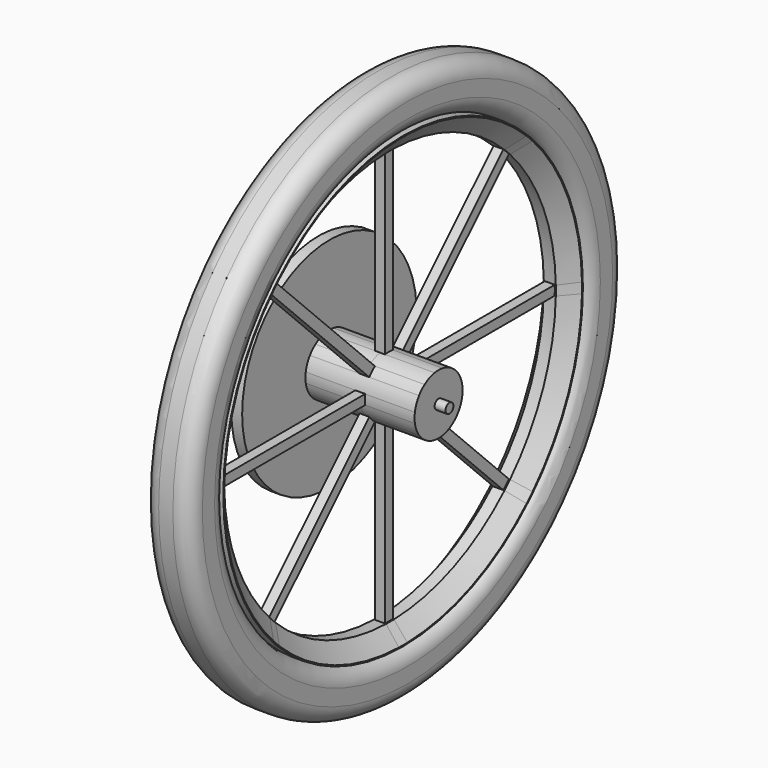
from build123d import *

# Parameters (mm, degrees)
F0_R       = 4.5
F1_DEPTH   = 60
F2_DEPTH   = 50
F3_DEPTH   = 4.5
F0_R_2     = 250
F0_R_3     = 206
F4_DEPTH   = 21.5
F5_DEPTH   = 17.5
F6_R       = 15
F7_SIZE2   = 12
F7_SIZE    = 15
F7_2_SIZE2 = 12
F7_2_SIZE  = 15
F8_R       = 100
F9_DEPTH   = 10
F10_R      = 4.5
F11_DEPTH  = 15


# Not quite as in the source:
# - a feature names something its author has since deleted; it is built from what else it names


with BuildPart() as f1:
    # F0 (on Right) → F1 (new body, symmetric)
    with BuildSketch(Plane.YZ):
        Circle(F0_R)
    extrude(amount=F1_DEPTH, both=True)

    # F0 (on Right) → F2 (join, symmetric)
    with BuildSketch(Plane.YZ):
        with BuildLine():
            ThreePointArc((27.5, 0), (27.4146857974, 2.1644866893), (27.1592725361, 4.3155434546))
            ThreePointArc((27.1592725361, 4.3155434546), (25.4422970206, 10.4374097514), (22.3653066086, 16.0013455779))
            ThreePointArc((22.3653066086, 16.0013455779), (19.4454364826, 19.4454364826), (16.0013455779, 22.3653066086))
            ThreePointArc((16.0013455779, 22.3653066086), (10.52379439, 25.4066871441), (4.5, 27.1293199325))
            ThreePointArc((4.5, 27.1293199325), (0, 27.5), (-4.5, 27.1293199325))
            ThreePointArc((-4.5, 27.1293199325), (-10.52379439, 25.4066871441), (-16.0013455779, 22.3653066086))
            ThreePointArc((-16.0013455779, 22.3653066086), (-19.4454364826, 19.4454364826), (-22.3653066086, 16.0013455779))
            ThreePointArc((-22.3653066086, 16.0013455779), (-25.4066871441, 10.52379439), (-27.1293199325, 4.5))
            ThreePointArc((-27.1293199325, 4.5), (-27.5, 0), (-27.1293199325, -4.5))
            ThreePointArc((-27.1293199325, -4.5), (-25.4066871441, -10.52379439), (-22.3653066086, -16.0013455779))
            ThreePointArc((-22.3653066086, -16.0013455779), (-19.4454364826, -19.4454364826), (-16.0013455779, -22.3653066086))
            ThreePointArc((-16.0013455779, -22.3653066086), (-10.52379439, -25.4066871441), (-4.5, -27.1293199325))
            ThreePointArc((-4.5, -27.1293199325), (0, -27.5), (4.5, -27.1293199325))
            ThreePointArc((4.5, -27.1293199325), (10.52379439, -25.4066871441), (16.0013455779, -22.3653066086))
            ThreePointArc((16.0013455779, -22.3653066086), (19.4454364826, -19.4454364826), (22.3653066086, -16.0013455779))
            ThreePointArc((22.3653066086, -16.0013455779), (25.4066871441, -10.52379439), (27.1293199325, -4.5))
            ThreePointArc((27.1293199325, -4.5), (27.4071733142, -2.2576206342), (27.5, 0))
        make_face()
        Circle(F0_R, mode=Mode.SUBTRACT)
    extrude(amount=F2_DEPTH, both=True)

    # F0 (on Right) → F3 (join, symmetric)
    with BuildSketch(Plane.YZ):
        with BuildLine():
            Line((4.5, 27.1293199325), (4.5, 189.9467030511))
            ThreePointArc((4.5, 189.9467030511), (0, 190), (-4.5, 189.9467030511))
            Line((-4.5, 189.9467030511), (-4.5, 27.1293199325))
            ThreePointArc((-4.5, 27.1293199325), (0, 27.5), (4.5, 27.1293199325))
        make_face()
        with BuildLine():
            Line((-16.0013455779, 22.3653066086), (-131.1306212762, 137.4945823068))
            ThreePointArc((-131.1306212762, 137.4945823068), (-134.3502884254, 134.3502884254), (-137.4945823068, 131.1306212762))
            Line((-137.4945823068, 131.1306212762), (-22.3653066086, 16.0013455779))
            ThreePointArc((-22.3653066086, 16.0013455779), (-19.4454364826, 19.4454364826), (-16.0013455779, 22.3653066086))
        make_face()
        with BuildLine():
            Line((-27.1293199325, 4.5), (-189.9467030511, 4.5))
            ThreePointArc((-189.9467030511, 4.5), (-190, 0), (-189.9467030511, -4.5))
            Line((-189.9467030511, -4.5), (-27.1293199325, -4.5))
            ThreePointArc((-27.1293199325, -4.5), (-27.5, 0), (-27.1293199325, 4.5))
        make_face()
        with BuildLine():
            ThreePointArc((-137.4945823068, -131.1306212762), (-134.3502884254, -134.3502884254), (-131.1306212762, -137.4945823068))
            Line((-131.1306212762, -137.4945823068), (-16.0013455779, -22.3653066086))
            ThreePointArc((-16.0013455779, -22.3653066086), (-19.4454364826, -19.4454364826), (-22.3653066086, -16.0013455779))
            Line((-22.3653066086, -16.0013455779), (-137.4945823068, -131.1306212762))
        make_face()
        with BuildLine():
            Line((22.3653066086, 16.0013455779), (137.4945823068, 131.1306212762))
            ThreePointArc((137.4945823068, 131.1306212762), (134.3502884254, 134.3502884254), (131.1306212762, 137.4945823068))
            Line((131.1306212762, 137.4945823068), (16.0013455779, 22.3653066086))
            ThreePointArc((16.0013455779, 22.3653066086), (19.4454364826, 19.4454364826), (22.3653066086, 16.0013455779))
        make_face()
        with BuildLine():
            ThreePointArc((131.1306212762, -137.4945823068), (134.3502884254, -134.3502884254), (137.4945823068, -131.1306212762))
            Line((137.4945823068, -131.1306212762), (22.3653066086, -16.0013455779))
            ThreePointArc((22.3653066086, -16.0013455779), (19.4454364826, -19.4454364826), (16.0013455779, -22.3653066086))
            Line((16.0013455779, -22.3653066086), (131.1306212762, -137.4945823068))
        make_face()
        with BuildLine():
            ThreePointArc((-4.5, -189.9467030511), (0, -190), (4.5, -189.9467030511))
            Line((4.5, -189.9467030511), (4.5, -27.1293199325))
            ThreePointArc((4.5, -27.1293199325), (0, -27.5), (-4.5, -27.1293199325))
            Line((-4.5, -27.1293199325), (-4.5, -189.9467030511))
        make_face()
        with BuildLine():
            ThreePointArc((189.9467030511, -4.5), (189.9866752956, -2.2501578036), (190, 0))
            ThreePointArc((190, 0), (189.9877454483, 2.1579109074), (189.9509833738, 4.3155434546))
            Line((189.9509833738, 4.3155434546), (27.1592725361, 4.3155434546))
            ThreePointArc((27.1592725361, 4.3155434546), (27.4146857974, 2.1644866893), (27.5, 0))
            ThreePointArc((27.5, 0), (27.4071733142, -2.2576206342), (27.1293199325, -4.5))
            Line((27.1293199325, -4.5), (189.9467030511, -4.5))
        make_face()
    extrude(amount=F3_DEPTH, both=True)

    # F8 (on face) → F9 (join)
    with BuildSketch(Plane(origin=(-50, 0, 0), x_dir=(0, -1, 0), z_dir=(-1, 0, 0))):
        Circle(F8_R)
    extrude(amount=F9_DEPTH)

    # F10 (on face) → F11 (join)
    with BuildSketch(Plane(origin=(-60, 0, 0), x_dir=(0, -1, 0), z_dir=(-1, 0, 0))):
        Circle(F10_R)
    extrude(amount=F11_DEPTH)


with BuildPart() as f4:
    # F0 (on Right) → F4 (new body, symmetric)
    with BuildSketch(Plane.YZ):
        Circle(F0_R_2)
        Circle(F0_R_3, mode=Mode.SUBTRACT)
    extrude(amount=F4_DEPTH, both=True)

    # F6
    f6_edges = [f4.edges().sort_by_distance(p)[0] for p in [
        (-21.5, -250, 0),
        (0, 250, 0),
        (21.5, -250, 0),
        (-21.5, -206, 0),
        (21.5, -206, 0),
    ]]
    fillet(f6_edges, radius=F6_R)


with BuildPart() as f5:
    # F0 (on Right) → F5 (new body, symmetric)
    with BuildSketch(Plane.YZ):
        Circle(F0_R_3)
        with BuildLine():
            ThreePointArc((189.9509833738, 4.3155434546), (189.9877454483, 2.1579109074), (190, 0))
            ThreePointArc((190, 0), (189.9866752956, -2.2501578036), (189.9467030511, -4.5))
            ThreePointArc((189.9467030511, -4.5), (175.5371111771, -72.7098521494), (137.4945823068, -131.1306212762))
            ThreePointArc((137.4945823068, -131.1306212762), (134.3502884254, -134.3502884254), (131.1306212762, -137.4945823068))
            ThreePointArc((131.1306212762, -137.4945823068), (72.7098521494, -175.5371111771), (4.5, -189.9467030511))
            ThreePointArc((4.5, -189.9467030511), (0, -190), (-4.5, -189.9467030511))
            ThreePointArc((-4.5, -189.9467030511), (-72.7098521494, -175.5371111771), (-131.1306212762, -137.4945823068))
            ThreePointArc((-131.1306212762, -137.4945823068), (-134.3502884254, -134.3502884254), (-137.4945823068, -131.1306212762))
            ThreePointArc((-137.4945823068, -131.1306212762), (-175.5371111771, -72.7098521494), (-189.9467030511, -4.5))
            ThreePointArc((-189.9467030511, -4.5), (-190, 0), (-189.9467030511, 4.5))
            ThreePointArc((-189.9467030511, 4.5), (-175.5371111771, 72.7098521494), (-137.4945823068, 131.1306212762))
            ThreePointArc((-137.4945823068, 131.1306212762), (-134.3502884254, 134.3502884254), (-131.1306212762, 137.4945823068))
            ThreePointArc((-131.1306212762, 137.4945823068), (-72.7098521494, 175.5371111771), (-4.5, 189.9467030511))
            ThreePointArc((-4.5, 189.9467030511), (0, 190), (4.5, 189.9467030511))
            ThreePointArc((4.5, 189.9467030511), (72.7098521494, 175.5371111771), (131.1306212762, 137.4945823068))
            ThreePointArc((131.1306212762, 137.4945823068), (134.3502884254, 134.3502884254), (137.4945823068, 131.1306212762))
            ThreePointArc((137.4945823068, 131.1306212762), (175.5723942188, 72.6246128271), (189.9509833738, 4.3155434546))
        make_face(mode=Mode.SUBTRACT)
    extrude(amount=F5_DEPTH, both=True)

    # F7
    f7_edges = [f5.edges().sort_by_distance(p)[0] for p in [
        (17.5, -190, 0),
    ]]
    f7_side = f5.faces().sort_by_distance((17.5, -200.17344, 0))[0]
    chamfer(f7_edges, length=F7_SIZE, length2=F7_SIZE2, reference=f7_side)

    # F7#2
    f7_2_edges = [f5.edges().sort_by_distance(p)[0] for p in [
        (-17.5, -190, 0),
    ]]
    f7_2_side = f5.faces().sort_by_distance((-17.5, -200.17344, 0))[0]
    chamfer(f7_2_edges, length=F7_2_SIZE, length2=F7_2_SIZE2, reference=f7_2_side)


solid = Compound([f1.part, f4.part, f5.part])
